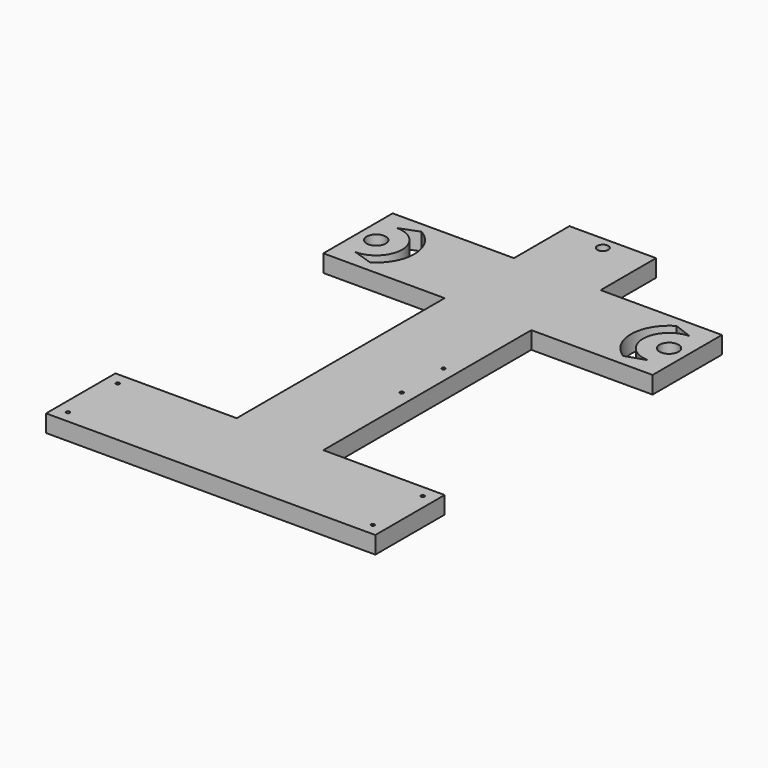
from build123d import *

# Parameters (mm, degrees)
F0_W      = 50
F0_H      = 150
F0_H_2    = 50
F0_W_2    = 70
F0_H_3    = 40
F1_DEPTH  = 10
F2_R      = 3.175
F3_DEPTH  = 10.001
F4_R      = 5.5
F5_DEPTH  = 10.001
F6_R      = 5.5
F7_DEPTH  = 10.001
F9_DEPTH  = 10.001
F11_D     = 2
F13_D     = 2
F14_R     = 5.5
F14_R_2   = 2.7
F15_DEPTH = 4
F16_DEPTH = 4


# Not quite as in the source:
# - a pattern or mirror of a feature is missing from the dataset's text; its kind, count and spacing are read off the source's solid
# - a feature names something its author has since deleted; it is built from what else it names


with BuildPart() as f1:
    # F0 (on Top) → F1 (new body)
    with BuildSketch(Plane.XY):
        Rectangle(F0_W, F0_H)
        with Locations((0, 100)):
            Rectangle(F0_W, F0_H_2)
        with Locations((60, 100)):
            Rectangle(F0_W_2, F0_H_2)
        with Locations((-60, 100)):
            Rectangle(F0_W_2, F0_H_2)
        with Locations((0, -100)):
            Rectangle(F0_W, F0_H_2)
        with Locations((60, -100)):
            Rectangle(F0_W_2, F0_H_2)
        with Locations((0, 145)):
            Rectangle(F0_W, F0_H_3)
        with Locations((-60, -100)):
            Rectangle(F0_W_2, F0_H_2)
    extrude(amount=F1_DEPTH)

    # F2 (on face) → F3 (cut, through all)
    with BuildSketch(Plane.XY.offset(10)):
        with Locations((0, 157.825)):
            Circle(F2_R)
    extrude(amount=-F3_DEPTH, mode=Mode.SUBTRACT)

    # F4 (on face) → F5 (cut, through all)
    with BuildSketch(Plane.XY.offset(10)):
        with Locations((-84.5, 100)):
            Circle(F4_R)
    extrude(amount=-F5_DEPTH, mode=Mode.SUBTRACT)

    # F6 (on face) → F7 (cut, through all)
    with BuildSketch(Plane.XY.offset(10)):
        with Locations((84.5, 100)):
            Circle(F6_R)
    extrude(amount=-F7_DEPTH, mode=Mode.SUBTRACT)

    # F8 (on face) → F9 (cut, through all)
    with BuildSketch(Plane.XY.offset(10)):
        with BuildLine():
            Line((73.023525645, 81.2305957373), (84.5, 85))
            ThreePointArc((84.5, 85), (69.5, 100), (84.5, 115))
            Line((84.5, 115), (73.5817295179, 119.0995122891))
            ThreePointArc((73.5817295179, 119.0995122891), (62.5023896916, 100.3242540951), (73.023525645, 81.2305957373))
        make_face()
        with BuildLine():
            Line((-84.5, 85), (-73.023525645, 81.2305957373))
            ThreePointArc((-73.023525645, 81.2305957373), (-62.5023896916, 100.3242540951), (-73.5817295179, 119.0995122891))
            Line((-73.5817295179, 119.0995122891), (-84.5, 115))
            ThreePointArc((-84.5, 115), (-69.5, 100), (-84.5, 85))
        make_face()
    extrude(amount=-F9_DEPTH, mode=Mode.SUBTRACT)

    # F11 (through all)
    with Locations(Plane.XY.offset(10)):
        with Locations((88, -82), (88, -118)):
            f11 = Hole(F11_D / 2)

    # F11_copies: F11 across plane
    add(f11.mirror(Plane(origin=(0, 0, 0), x_dir=(0, 0, -1), z_dir=(-1, 0, 0))), mode=Mode.SUBTRACT)

    # F13 (through all)
    with Locations(Plane(origin=(0, 0, 0), x_dir=(1, 0, 0), z_dir=(0, 0, -1))):
        with Locations((17.5, -21), (17.5, 9)):
            Hole(F13_D / 2)

    # F14 (on Top) → F15 (join)
    with BuildSketch(Plane.XY):
        with Locations((84.5, 100)):
            Circle(F14_R)
        with Locations((84.5, 100)):
            Circle(F14_R_2, mode=Mode.SUBTRACT)
        with Locations((-84.5, 100)):
            Circle(F14_R)
        with Locations((-84.5, 100)):
            Circle(F14_R_2, mode=Mode.SUBTRACT)
    extrude(amount=F15_DEPTH)

    # F14 (on Top) → F16 (join)
    with BuildSketch(Plane.XY):
        with Locations((84.5, 100)):
            Circle(F14_R)
        with Locations((84.5, 100)):
            Circle(F14_R_2, mode=Mode.SUBTRACT)
        with Locations((-84.5, 100)):
            Circle(F14_R)
        with Locations((-84.5, 100)):
            Circle(F14_R_2, mode=Mode.SUBTRACT)
    extrude(amount=F16_DEPTH)


solid = f1.part
